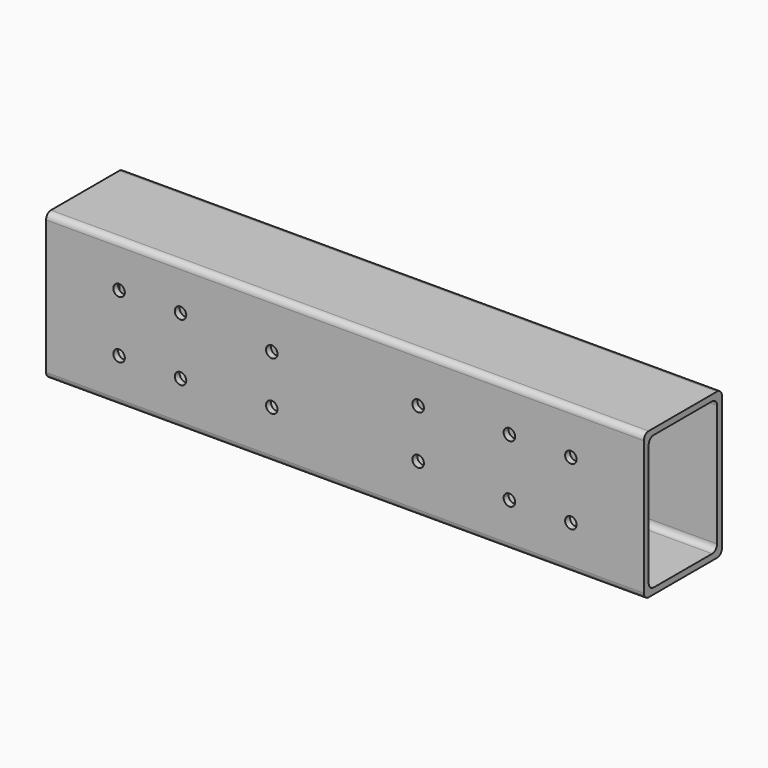
from build123d import *

# Parameters (mm, degrees)
F0_W     = 50.8
F0_H     = 76.2
F0_W_2   = 44.45
F0_H_2   = 69.85
F2_DEPTH = 311.15
F3_R     = 3.175
F4_R     = 3
F5_DEPTH = 25.4
F6_DEPTH = 25.4


# Not quite as in the source:
# - a variable given as a bare number and used for a length is read in inches; the dataset says mm whatever the document's units were


with BuildPart() as f2:
    # F0 (on Right) → F2 (new body)
    with BuildSketch(Plane.YZ):
        Rectangle(F0_W, F0_H)
        Rectangle(F0_W_2, F0_H_2, mode=Mode.SUBTRACT)
    extrude(amount=F2_DEPTH)

    # F3
    f3_edges = [f2.edges().sort_by_distance(p)[0] for p in [
        (155.575, -25.4, 38.1),
        (155.575, -22.225, 34.925),
        (155.575, 22.225, 34.925),
        (155.575, 25.4, 38.1),
        (155.575, 25.4, -38.1),
        (155.575, -25.4, -38.1),
        (155.575, 22.225, -34.925),
        (155.575, -22.225, -34.925),
    ]]
    fillet(f3_edges, radius=F3_R)

    # F4 (on face) → F5 (cut)
    with BuildSketch(Plane.XZ.offset(25.4)):
        with Locations((37.975, 15)):
            Circle(F4_R)
        with Locations((69.975, 15)):
            Circle(F4_R)
        with Locations((69.975, -15)):
            Circle(F4_R)
        with Locations((37.975, -15)):
            Circle(F4_R)
        with Locations((241.175, 15)):
            Circle(F4_R)
        with Locations((273.175, 15)):
            Circle(F4_R)
        with Locations((273.175, -15)):
            Circle(F4_R)
        with Locations((241.175, -15)):
            Circle(F4_R)
    extrude(amount=-F5_DEPTH, mode=Mode.SUBTRACT)

    # F4 (on face) → F6 (cut)
    with BuildSketch(Plane.XZ.offset(25.4)):
        with Locations((117.475, 12.7)):
            Circle(F4_R)
        with Locations((117.475, -12.7)):
            Circle(F4_R)
        with Locations((193.675, -12.7)):
            Circle(F4_R)
        with Locations((193.675, 12.7)):
            Circle(F4_R)
    extrude(amount=-F6_DEPTH, mode=Mode.SUBTRACT)


solid = f2.part
